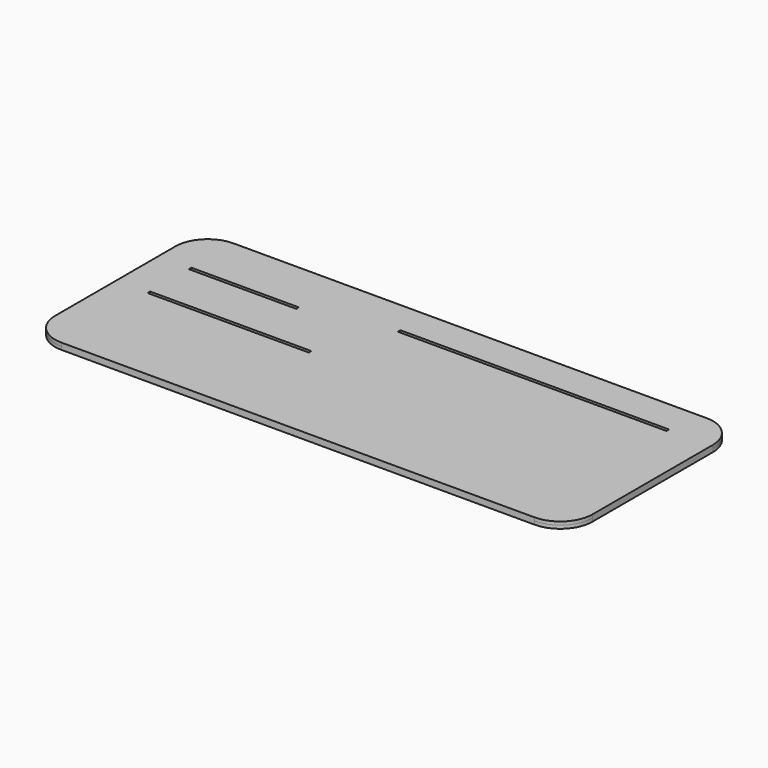
from build123d import *

# Parameters (mm, degrees)
F0_W        = 500
F0_H        = 200
F1_DEPTH    = 3
F2_R        = 30
F3_W        = 100
F3_H        = 3
F3_W_2      = 150
F3_W_3      = 250
F4_DEPTH    = 3
F5_W        = 500
F5_H        = 200
F6_DEPTH    = 3
F7_T1_DEPTH = 152.9995000008


# Not quite as in the source:
# - a fillet or chamfer that OpenCascade refuses, or shapes differently, is made with other operations: its cross-section is extruded or revolved along the edge and cut away or added


with BuildPart() as f1:
    # F0 (on Top) → F1 (new body)
    with BuildSketch(Plane.XY):
        Rectangle(F0_W, F0_H)
    extrude(amount=F1_DEPTH)

    # F2
    f2_edges = [f1.edges().sort_by_distance(p)[0] for p in [
        (-250, -100, 1.5),
        (250, 100, 1.5),
        (-250, 100, 1.5),
        (250, -100, 1.5),
    ]]
    fillet(f2_edges, radius=F2_R)

    # F3 (on face) → F4 (cut)
    with BuildSketch(Plane.XY.offset(3)):
        with Locations((-170, 49.5)):
            Rectangle(F3_W, F3_H)
        with Locations((-145, 1.5)):
            Rectangle(F3_W_2, F3_H)
        with Locations((85, 67.5)):
            Rectangle(F3_W_3, F3_H)
    extrude(amount=-F4_DEPTH, mode=Mode.SUBTRACT)

    # F5 (on face) → F6 (join)
    with BuildSketch(Plane(origin=(0, 0, 0), x_dir=(1, 0, 0), z_dir=(0, 0, -1))):
        Rectangle(F5_W, F5_H)
    extrude(amount=F6_DEPTH)

    # F7: fillet of radius 30 on 4 edges, made by hand

    # F7_s2 → F7_t1 (cut)
    with BuildSketch(Plane.XY.offset(-77.9997500004)):
        with BuildLine():
            ThreePointArc((-220.0001, -100.0001), (-241.2133034356, -91.2133034356), (-250.0001, -70.0001))
            Line((-250.0001, -70.0001), (-250.6001, -70.0001))
            ThreePointArc((-250.6001, -70.0001), (-250.6, -85.00005), (-250.6, -100))
            Line((-250.6, -100), (-250, -100.6))
            ThreePointArc((-250, -100.6), (-235.00005, -100.6), (-220.0001, -100.6001))
            Line((-220.0001, -100.6001), (-220.0001, -100.0001))
        make_face()
        with BuildLine():
            ThreePointArc((-250.0001, 70.0001), (-241.2133034356, 91.2133034356), (-220.0001, 100.0001))
            Line((-220.0001, 100.0001), (-220.0001, 100.6001))
            ThreePointArc((-220.0001, 100.6001), (-235.00005, 100.6), (-250, 100.6))
            Line((-250, 100.6), (-250.6, 100))
            ThreePointArc((-250.6, 100), (-250.6, 85.00005), (-250.6001, 70.0001))
            Line((-250.6001, 70.0001), (-250.0001, 70.0001))
        make_face()
        with BuildLine():
            ThreePointArc((250.0001, 70.0001), (241.2133034356, 91.2133034356), (220.0001, 100.0001))
            Line((220.0001, 100.0001), (220.0001, 100.6001))
            ThreePointArc((220.0001, 100.6001), (235.00005, 100.6), (250, 100.6))
            Line((250, 100.6), (250.6, 100))
            ThreePointArc((250.6, 100), (250.6, 85.00005), (250.6001, 70.0001))
            Line((250.6001, 70.0001), (250.0001, 70.0001))
        make_face()
        with BuildLine():
            ThreePointArc((220.0001, -100.0001), (241.2133034356, -91.2133034356), (250.0001, -70.0001))
            Line((250.0001, -70.0001), (250.6001, -70.0001))
            ThreePointArc((250.6001, -70.0001), (250.6, -85.00005), (250.6, -100))
            Line((250.6, -100), (250, -100.6))
            ThreePointArc((250, -100.6), (235.00005, -100.6), (220.0001, -100.6001))
            Line((220.0001, -100.6001), (220.0001, -100.0001))
        make_face()
    extrude(amount=F7_T1_DEPTH, mode=Mode.SUBTRACT)


solid = f1.part
